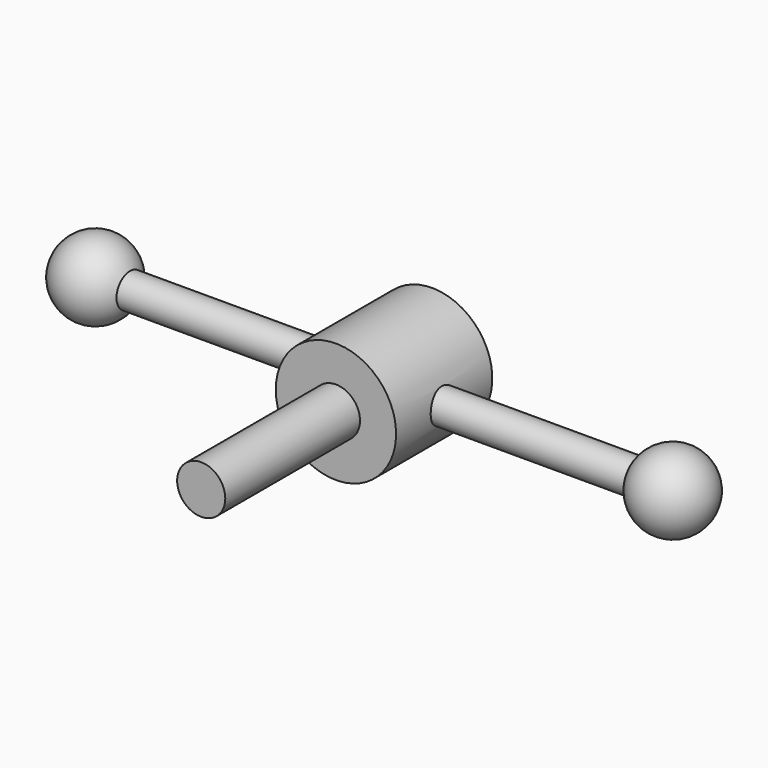
from build123d import *

# Parameters (mm, degrees)
F0_R     = 6.35
F1_DEPTH = 44.45
F2_R     = 15.875
F2_R_2   = 6.35
F3_DEPTH = 31.75


with BuildPart() as f1:
    # F0 (on Front) → F1 (new body)
    with BuildSketch(Plane.XZ):
        Circle(F0_R)
    extrude(amount=F1_DEPTH)

    # F2 (on face) → F3 (join)
    with BuildSketch(Plane(origin=(0, 0, 0), x_dir=(-1, 0, 0), z_dir=(0, 1, 0))):
        Circle(F2_R)
        Circle(F2_R_2, mode=Mode.SUBTRACT)
        Circle(F2_R_2)
    extrude(amount=F3_DEPTH)

    # F4 (on Top) → F5 (revolve)
    with BuildSketch(Plane.XY):
        with BuildLine():
            ThreePointArc((-67.0639409481, 20.32), (-78.4807060346, 25.7757060346), (-86.36, 15.875))
            Line((-86.36, 15.875), (-66.04, 15.875))
            ThreePointArc((-66.04, 15.875), (-66.2992939654, 18.1557060346), (-67.0639409481, 20.32))
        make_face()
        with BuildLine():
            ThreePointArc((-67.0639409481, 20.32), (-66.2992939654, 18.1557060346), (-66.04, 15.875))
            Line((-66.04, 15.875), (66.04, 15.875))
            ThreePointArc((66.04, 15.875), (66.2992939654, 18.1557060346), (67.0639409481, 20.32))
            Line((67.0639409481, 20.32), (-67.0639409481, 20.32))
        make_face()
        with BuildLine():
            ThreePointArc((67.0639409481, 20.32), (66.2992939654, 18.1557060346), (66.04, 15.875))
            Line((66.04, 15.875), (86.36, 15.875))
            ThreePointArc((86.36, 15.875), (78.4807060346, 25.7757060346), (67.0639409481, 20.32))
        make_face()
    revolve(axis=Axis((0, 15.875, 0), (1, 0, 0)))


solid = f1.part
